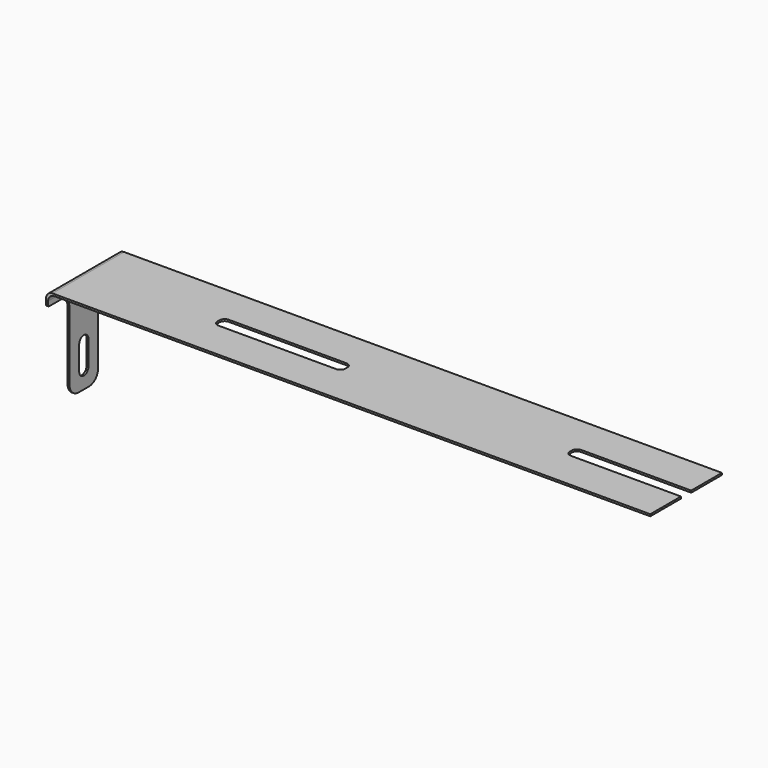
from build123d import *

# Parameters (mm, degrees)
F0_W     = 4
F0_H     = 3
F1_DEPTH = 0.15
F2_DEPTH = 1.9
F3_W     = 0.15
F3_H     = 7
F4_DEPTH = 8
F6_DEPTH = 25
F7_R     = 0.5


# Not quite as in the source:
# - a feature names something its author has since deleted; it is built from what else it names


with BuildPart() as f1:
    # F0 (on Top) → F1 (new body)
    with BuildSketch(Plane.XY):
        with BuildLine():
            Line((13.775, -0.5), (13.775, -3.5))
            Line((13.775, -3.5), (27.55, -3.5))
            Line((27.55, -3.5), (41.325, -3.5))
            Line((41.325, -3.5), (41.325, -0.5))
            Line((41.325, -0.5), (36.725, -0.5))
            ThreePointArc((36.725, -0.5), (36.4421572875, -0.3828427125), (36.325, -0.1))
            Line((36.325, -0.1), (36.325, 0.1))
            ThreePointArc((36.325, 0.1), (36.4421572875, 0.3828427125), (36.725, 0.5))
            Line((36.725, 0.5), (41.325, 0.5))
            Line((41.325, 0.5), (41.325, 3.5))
            Line((41.325, 3.5), (27.55, 3.5))
            Line((27.55, 3.5), (13.775, 3.5))
            Line((13.775, 3.5), (13.775, 0.5))
            Line((13.775, 0.5), (18.375, 0.5))
            ThreePointArc((18.375, 0.5), (18.6578427125, 0.3828427125), (18.775, 0.1))
            Line((18.775, 0.1), (18.775, -0.1))
            ThreePointArc((18.775, -0.1), (18.6578427125, -0.3828427125), (18.375, -0.5))
            Line((18.375, -0.5), (13.775, -0.5))
        make_face()
        with Locations((43.325, 2)):
            Rectangle(F0_W, F0_H)
        with BuildLine():
            Line((0, 3.5), (0, -3.5))
            Line((0, -3.5), (13.775, -3.5))
            Line((13.775, -3.5), (13.775, -0.5))
            Line((13.775, -0.5), (9.175, -0.5))
            ThreePointArc((9.175, -0.5), (8.8921572875, -0.3828427125), (8.775, -0.1))
            Line((8.775, -0.1), (8.775, 0.1))
            ThreePointArc((8.775, 0.1), (8.8921572875, 0.3828427125), (9.175, 0.5))
            Line((9.175, 0.5), (13.775, 0.5))
            Line((13.775, 0.5), (13.775, 3.5))
            Line((13.775, 3.5), (0, 3.5))
        make_face()
        with Locations((43.325, -2)):
            Rectangle(F0_W, F0_H)
    extrude(amount=F1_DEPTH)

    # F2 (add): a face of the model
    f2_faces = [f1.faces().sort_by_distance(p)[0] for p in [
        (0, 0, 0.075),
    ]]
    extrude(f2_faces, amount=F2_DEPTH)

    # F3 (on face) → F4 (join)
    with BuildSketch(Plane(origin=(0, 0, 0), x_dir=(1, 0, 0), z_dir=(0, 0, -1))):
        with Locations((-1.825, 0)):
            Rectangle(F3_W, F3_H)
    extrude(amount=F4_DEPTH)

    # F5 (on face) → F6 (cut)
    with BuildSketch(Plane(origin=(-1.9, 0, 0), x_dir=(0, -1, 0), z_dir=(-1, 0, 0))):
        with BuildLine():
            Line((-3.5, -8), (-0.5, -8))
            ThreePointArc((-0.5, -8), (-1.1363961031, -7.7363961031), (-1.4, -7.1))
            Line((-1.4, -7.1), (-1.4, -1.8))
            ThreePointArc((-1.4, -1.8), (-1.6636038969, -1.1636038969), (-2.3, -0.9))
            Line((-2.3, -0.9), (-3.4, -0.9))
            ThreePointArc((-3.4, -0.9), (-3.4707106781, -0.8707106781), (-3.5, -0.8))
            Line((-3.5, -0.8), (-3.5, -8))
        make_face()
        with BuildLine():
            ThreePointArc((1.4, -7.1), (1.1363961031, -7.7363961031), (0.5, -8))
            Line((0.5, -8), (3.5, -8))
            Line((3.5, -8), (3.5, -0.8))
            ThreePointArc((3.5, -0.8), (3.4707106781, -0.8707106781), (3.4, -0.9))
            Line((3.4, -0.9), (2.3, -0.9))
            ThreePointArc((2.3, -0.9), (1.6636038969, -1.1636038969), (1.4, -1.8))
            Line((1.4, -1.8), (1.4, -7.1))
        make_face()
        with BuildLine():
            ThreePointArc((-0.45, -6.6), (0, -7.05), (0.45, -6.6))
            ThreePointArc((0.45, -6.6), (0, -6.15), (-0.45, -6.6))
        make_face()
        with BuildLine():
            ThreePointArc((-0.45, -6.6), (0, -6.15), (0.45, -6.6))
            Line((0.45, -6.6), (0.45, -4.7))
            ThreePointArc((0.45, -4.7), (0, -5.15), (-0.45, -4.7))
            Line((-0.45, -4.7), (-0.45, -6.6))
        make_face()
        with BuildLine():
            ThreePointArc((-0.45, -4.7), (0, -5.15), (0.45, -4.7))
            ThreePointArc((0.45, -4.7), (0, -4.25), (-0.45, -4.7))
        make_face()
    extrude(amount=-F6_DEPTH, mode=Mode.SUBTRACT)

    # F7
    f7_edges = [f1.edges().sort_by_distance(p)[0] for p in [
        (-1.9, 0, 0.15),
        (-1.75, 0, 0),
    ]]
    fillet(f7_edges, radius=F7_R)


solid = f1.part
